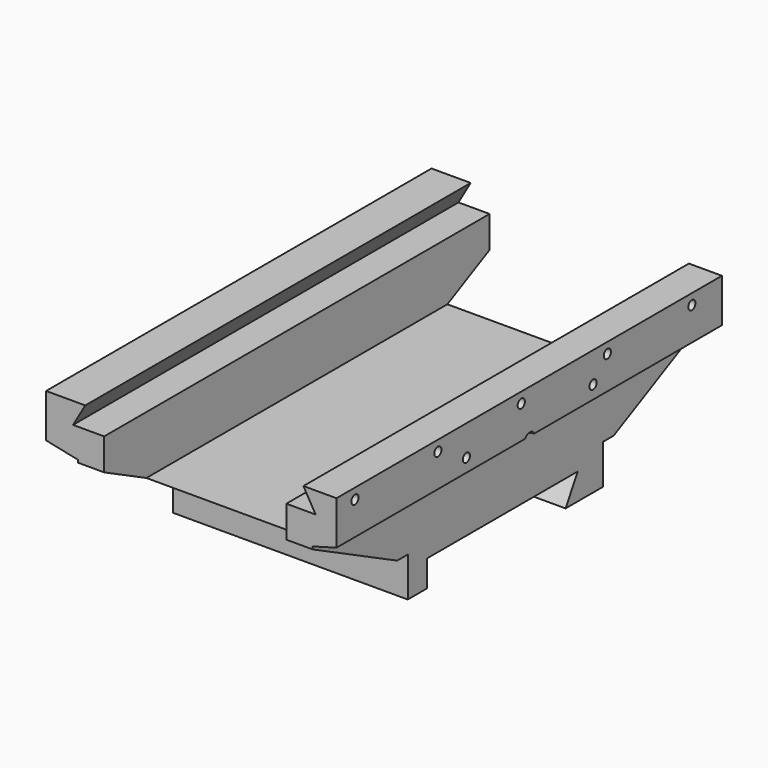
from build123d import *

# Parameters (mm, degrees)
F1_DEPTH  = 182.5
F3_DEPTH  = 200
F5_DEPTH  = 200
F7_DEPTH  = 220.001
F8_W      = 138
F8_H      = 20
F8_H_2    = 24
F9_DEPTH  = 365.001
F12_DEPTH = 35
F10_R     = 3.4
F14_DEPTH = 22.3866406461
F13_R     = 3.4
F15_DEPTH = 25
F16_DEPTH = 25


with BuildPart() as f1:
    # F0 (on Front) → F1 (new body, symmetric)
    with BuildSketch(Plane.XZ):
        Polygon((110, 0), (-110, 0), (-110, -33), (-86, -38), (-86, -110), (92, -110), (92, -38), (110, -33), align=None)
    extrude(amount=F1_DEPTH, both=True)

    # F2 (on Front) → F3 (cut, symmetric)
    with BuildSketch(Plane.XZ):
        Polygon((84.9585481157, 0), (-80.3397459622, 0), (-89.5773502692, -16), (94.1961524227, -16), align=None)
    extrude(amount=F3_DEPTH, both=True, mode=Mode.SUBTRACT)

    # F4 (on Right) → F5 (cut, symmetric)
    with BuildSketch(Plane.YZ):
        Polygon((-74.5, -90), (-74.5, -110), (56.9529946162, -110), (68.5, -90), align=None)
    extrude(amount=F5_DEPTH, both=True, mode=Mode.SUBTRACT)

    # F6 (on face) → F7 (cut, through all)
    with BuildSketch(Plane.YZ.offset(110)):
        Polygon((-102.5, -80), (-182.5, -40), (-182.5, -150), (-92.5, -150), (-92.5, -80), align=None)
        Polygon((182.5, -150), (182.5, -40), (102.5, -80), (92.5, -80), (92.5, -150), align=None)
    extrude(amount=-F7_DEPTH, mode=Mode.SUBTRACT)

    # F8 (on face) → F9 (cut, through all)
    with BuildSketch(Plane.XZ.offset(182.5)):
        with Locations((3, -50)):
            Rectangle(F8_W, F8_H)
        with Locations((3, -28)):
            Rectangle(F8_W, F8_H_2)
    extrude(amount=-F9_DEPTH, mode=Mode.SUBTRACT)

    # F11 (on face) → F12 (cut)
    with BuildSketch(Plane.YZ.offset(110)):
        with BuildLine():
            Line((-3.9452221542, -33), (4.9452221542, -33))
            ThreePointArc((4.9452221542, -33), (0.5, -30.4), (-3.9452221542, -33))
        make_face()
        with BuildLine():
            ThreePointArc((-3.9452221542, -33), (-0.7921623377, -40.4335906289), (5.6, -35.5))
            ThreePointArc((5.6, -35.5), (5.4335906289, -34.2078376623), (4.9452221542, -33))
            Line((4.9452221542, -33), (-3.9452221542, -33))
        make_face()
    extrude(amount=-F12_DEPTH, mode=Mode.SUBTRACT)

    # F10 (on face) → F14 (cut, through all)
    with BuildSketch(Plane.YZ.offset(110)):
        with Locations((-165, -8)):
            Circle(F10_R)
        with Locations((-86.5, -8)):
            Circle(F10_R)
        with Locations((-7.5, -8)):
            Circle(F10_R)
        with Locations((74, -8)):
            Circle(F10_R)
        with Locations((154, -8)):
            Circle(F10_R)
    extrude(amount=-F14_DEPTH, mode=Mode.SUBTRACT)

    # F13 (on face) → F15 (cut)
    with BuildSketch(Plane.YZ.offset(110)):
        with Locations((-59.5, -23)):
            Circle(F13_R)
        with Locations((60.5, -23)):
            Circle(F13_R)
    extrude(amount=-F15_DEPTH, mode=Mode.SUBTRACT)

    # F13 (on face) → F16 (cut)
    with BuildSketch(Plane.YZ.offset(110)):
        with Locations((-59.5, -23)):
            Circle(F13_R)
        with Locations((60.5, -23)):
            Circle(F13_R)
    extrude(amount=-F16_DEPTH, mode=Mode.SUBTRACT)


solid = f1.part
